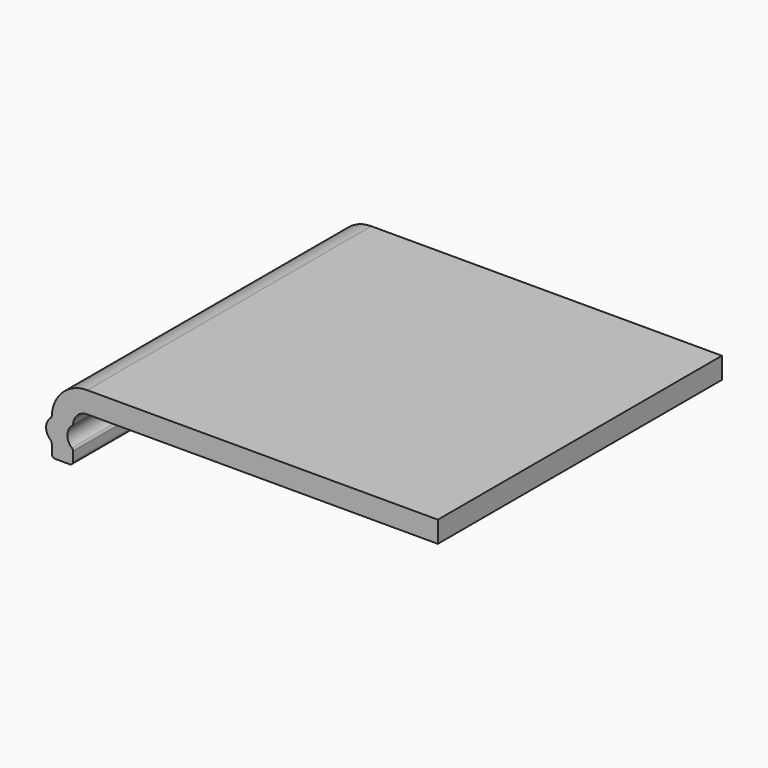
from build123d import *

# Parameters (mm, degrees)
F1_DEPTH = 25
F2_R     = 0.25


with BuildPart() as f1:
    # F0 (on Front) → F1 (new body)
    with BuildSketch(Plane.XZ):
        with BuildLine():
            Line((-24.683436538, 0), (0, 0))
            Line((0, 0), (0, 1.5))
            Line((0, 1.5), (-24.683436538, 1.5))
            ThreePointArc((-24.683436538, 1.5), (-26.451203491, 0.767766953), (-27.183436538, -1))
            ThreePointArc((-27.183436538, -1), (-27.583436538, -1.7483314774), (-27.183436538, -2.4966629547))
            Line((-27.183436538, -2.4966629547), (-27.183436538, -3.4966629547))
            Line((-27.183436538, -3.4966629547), (-25.683436538, -3.4966629547))
            Line((-25.683436538, -3.4966629547), (-25.683436538, -2.4966629547))
            ThreePointArc((-25.683436538, -2.4966629547), (-26.083436538, -1.7483314774), (-25.683436538, -1))
            ThreePointArc((-25.683436538, -1), (-25.3905433192, -0.2928932188), (-24.683436538, 0))
        make_face()
    extrude(amount=F1_DEPTH)

    # F2
    f2_edges = [f1.edges().sort_by_distance(p)[0] for p in [
        (-27.183437, -12.5, -3.496663),
        (-25.683437, -12.5, -3.496663),
        (-25.683437, -12.5, -2.496663),
        (-25.683437, -12.5, -1),
        (-27.183437, -12.5, -2.496663),
        (-27.183437, -12.5, -1),
    ]]
    fillet(f2_edges, radius=F2_R)


solid = f1.part
